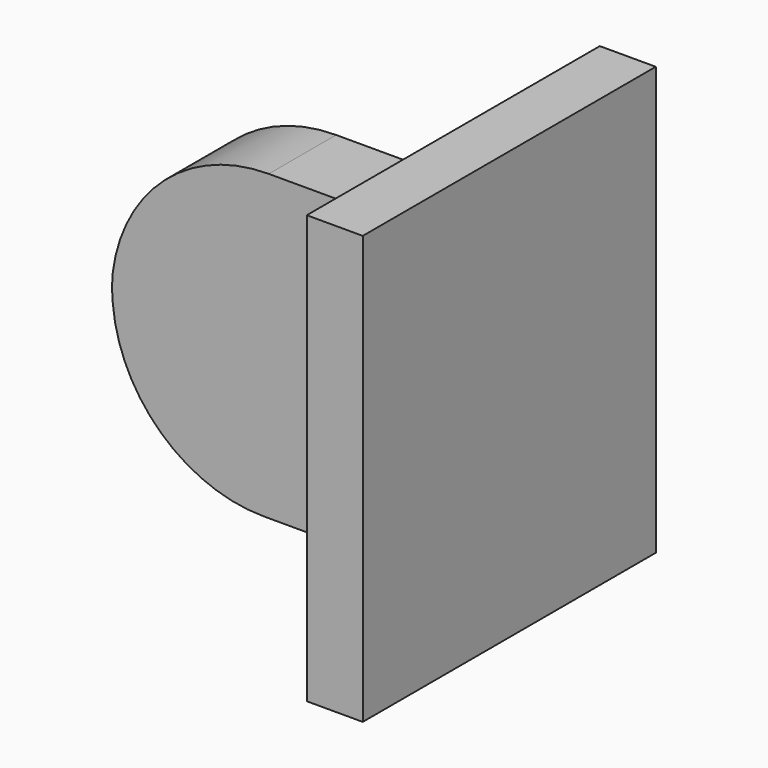
from build123d import *

# Parameters (mm, degrees)
F1_DEPTH    = 245.36945
F2_DEPTH    = 203.2
F3_W        = 163.0290746689
F3_H        = 1246.3291883469
F4_DEPTH    = 635
F5_DEPTH    = 431.8
F6_T1_DEPTH = 2516.4554829813
F7_T1_DEPTH = 2441.5924956103


# Not quite as in the source:
# - a fillet or chamfer that OpenCascade refuses, or shapes differently, is made with other operations: its cross-section is extruded or revolved along the edge and cut away or added


with BuildPart() as f1:
    # F0 (on Front) → F1 (new body)
    with BuildSketch(Plane.XZ):
        with BuildLine():
            Line((-437.8447532654, -40.3878050825), (-437.8447532654, 40.3878050825))
            ThreePointArc((-437.8447532654, 40.3878050825), (-439.703539628, 0), (-437.8447532654, -40.3878050825))
        make_face()
        with BuildLine():
            Line((-437.8447532654, 439.703539628), (-437.8447532654, 40.3878050825))
            Line((-437.8447532654, 40.3878050825), (-437.8447532654, -40.3878050825))
            Line((-437.8447532654, -40.3878050825), (-437.8447532654, -443.3148503304))
            Line((-437.8447532654, -443.3148503304), (0, -443.3148503304))
            Line((0, -443.3148503304), (0, -127))
            ThreePointArc((0, -127), (-127, 0), (0, 127))
            Line((0, 127), (0, 439.703539628))
            Line((0, 439.703539628), (-437.8447532654, 439.703539628))
        make_face()
        with BuildLine():
            Line((440.1807188988, 439.703539628), (0, 439.703539628))
            Line((0, 439.703539628), (0, 127))
            ThreePointArc((0, 127), (89.8025612107, 89.8025612107), (127, 0))
            ThreePointArc((127, 0), (89.8025612107, -89.8025612107), (0, -127))
            Line((0, -127), (0, -443.3148503304))
            Line((0, -443.3148503304), (440.1807188988, -443.3148503304))
            Line((440.1807188988, -443.3148503304), (440.1807188988, 439.703539628))
        make_face()
        with BuildLine():
            Line((0, -127), (0, 127))
            ThreePointArc((0, 127), (-127, 0), (0, -127))
        make_face()
        with BuildLine():
            ThreePointArc((127, 0), (89.8025612107, 89.8025612107), (0, 127))
            Line((0, 127), (0, -127))
            ThreePointArc((0, -127), (89.8025612107, -89.8025612107), (127, 0))
        make_face()
    extrude(amount=F1_DEPTH)

    # F0 (on Front) → F2 (join)
    with BuildSketch(Plane.XZ):
        with BuildLine():
            Line((0, -127), (0, 127))
            ThreePointArc((0, 127), (-127, 0), (0, -127))
        make_face()
        with BuildLine():
            ThreePointArc((127, 0), (89.8025612107, 89.8025612107), (0, 127))
            Line((0, 127), (0, -127))
            ThreePointArc((0, -127), (89.8025612107, -89.8025612107), (127, 0))
        make_face()
    extrude(amount=-F2_DEPTH)

    # F3 (on Front) → F4 (join)
    with BuildSketch(Plane.XZ):
        with Locations((520.3551054001, 6.3239336014)):
            Rectangle(F3_W, F3_H)
    extrude(amount=F4_DEPTH)

    # F3 (on Front) → F5 (join)
    with BuildSketch(Plane.XZ):
        with Locations((520.3551054001, 6.3239336014)):
            Rectangle(F3_W, F3_H)
    extrude(amount=-F5_DEPTH)

    # F6: fillet of radius 457.9913774748 on 1 edges, made by hand

    # F6_s2 → F6_t1 (cut)
    with BuildSketch(Plane.XZ.offset(-1135.5430164906)):
        with BuildLine():
            ThreePointArc((16.3724533309, 439.703539628), (-286.0206379525, 325.6809400755), (-437.8447532654, 40.3878050825))
            Line((-437.8447532654, 40.3878050825), (-437.8447532654, 439.703539628))
            Line((-437.8447532654, 439.703539628), (16.3724533309, 439.703539628))
        make_face()
    extrude(amount=F6_T1_DEPTH, mode=Mode.SUBTRACT)

    # F7: fillet of radius 440.8813389734 on 1 edges, made by hand

    # F7_s2 → F7_t1 (cut)
    with BuildSketch(Plane.XZ.offset(-1098.1115228051)):
        with BuildLine():
            ThreePointArc((-437.8447532654, -40.3878050825), (-296.6295178781, -327.3255664249), (1.3998558567, -443.3148503304))
            Line((1.3998558567, -443.3148503304), (-437.8447532654, -443.3148503304))
            Line((-437.8447532654, -443.3148503304), (-437.8447532654, -40.3878050825))
        make_face()
    extrude(amount=F7_T1_DEPTH, mode=Mode.SUBTRACT)


solid = f1.part
